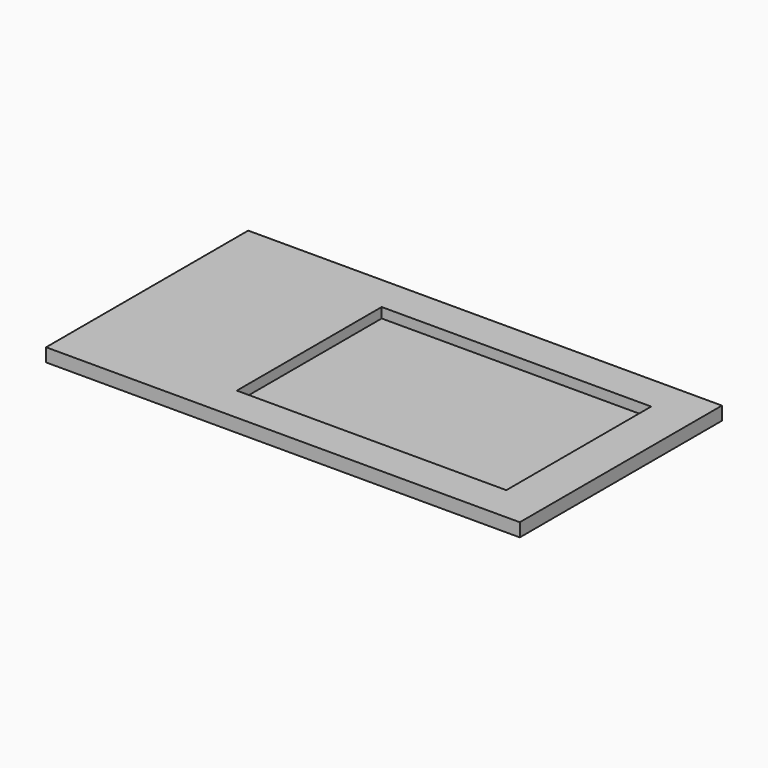
from build123d import *

# Parameters (mm, degrees)
F0_W     = 225
F0_H     = 120
F1_DEPTH = 6.35
F2_W     = 128
F2_H     = 86
F3_DEPTH = 4.8


# Not quite as in the source:
# - a length typed as a fraction of an inch, garbled in the dataset ("3 / 203.2 mm" for 3/8 in), is restored


with BuildPart() as f1:
    # F0 (on Top) → F1 (new body)
    with BuildSketch(Plane.XY):
        Rectangle(F0_W, F0_H)
    extrude(amount=F1_DEPTH)

    # F2 (on face) → F3 (cut)
    with BuildSketch(Plane.XY.offset(6.35)):
        with Locations((28.5, 0)):
            Rectangle(F2_W, F2_H)
    extrude(amount=-F3_DEPTH, mode=Mode.SUBTRACT)


solid = f1.part
